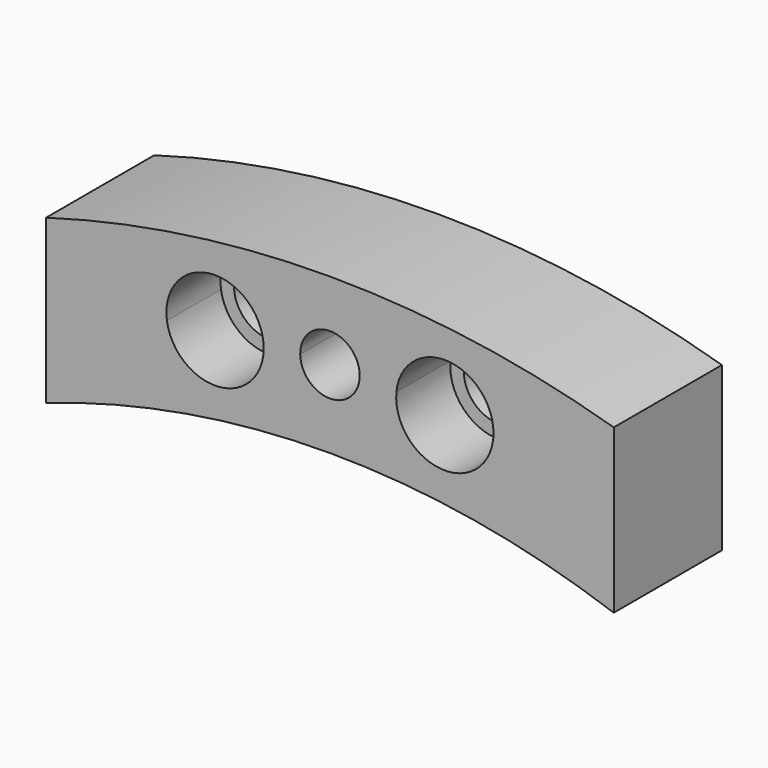
from build123d import *

# Parameters (mm, degrees)
F1_DEPTH = 50
F2_DEPTH = 25


with BuildPart() as f1:
    # F0 (on Front) → F1 (new body)
    with BuildSketch(Plane.XZ):
        with BuildLine():
            ThreePointArc((60.3004275437, 340.9588258691), (82.833452945, 336.1958976151), (105, 329.9455447494))
            Line((105, 329.9455447494), (105, 360))
            ThreePointArc((105, 360), (0, 375), (-105, 360))
            Line((-105, 360), (-105, 329.9455447494))
            ThreePointArc((-105, 329.9455447494), (-82.833452945, 336.1958976151), (-60.3004275437, 340.9588258691))
            ThreePointArc((-60.3004275437, 340.9588258691), (-44.7093862816, 361.4956891559), (-24.5847162741, 345.3761054643))
            ThreePointArc((-24.5847162741, 345.3761054643), (-17.7950983093, 345.7924189108), (-10.9986121712, 346.0752707581))
            ThreePointArc((-10.9986121712, 346.0752707581), (-0.0873673767, 357.2496530373), (11, 346.25))
            ThreePointArc((11, 346.25), (10.9996530373, 346.1626326233), (10.9986121712, 346.0752707581))
            ThreePointArc((10.9986121712, 346.0752707581), (17.7950983093, 345.7924189108), (24.5847162741, 345.3761054643))
            ThreePointArc((24.5847162741, 345.3761054643), (43.3731818064, 361.6106063163), (60.5, 343.6317978593))
            ThreePointArc((60.5, 343.6317978593), (60.4500375457, 342.2915918653), (60.3004275437, 340.9588258691))
        make_face()
        with BuildLine():
            ThreePointArc((-105, 299.635194862), (0, 317.5), (105, 299.635194862))
            Line((105, 299.635194862), (105, 329.9455447494))
            ThreePointArc((105, 329.9455447494), (82.833452945, 336.1958976151), (60.3004275437, 340.9588258691))
            ThreePointArc((60.3004275437, 340.9588258691), (40.2906137184, 325.7679065626), (24.5847162741, 345.3761054643))
            ThreePointArc((24.5847162741, 345.3761054643), (17.7950983093, 345.7924189108), (10.9986121712, 346.0752707581))
            ThreePointArc((10.9986121712, 346.0752707581), (0, 335.25), (-10.9986121712, 346.0752707581))
            ThreePointArc((-10.9986121712, 346.0752707581), (-17.7950983093, 345.7924189108), (-24.5847162741, 345.3761054643))
            ThreePointArc((-24.5847162741, 345.3761054643), (-24.521191543, 344.5049796657), (-24.5, 343.6317978593))
            ThreePointArc((-24.5, 343.6317978593), (-41.159794006, 325.6817603135), (-60.3004275437, 340.9588258691))
            ThreePointArc((-60.3004275437, 340.9588258691), (-82.833452945, 336.1958976151), (-105, 329.9455447494))
            Line((-105, 329.9455447494), (-105, 299.635194862))
        make_face()
        with BuildLine():
            ThreePointArc((-24.5847162741, 345.3761054643), (-44.7093862816, 361.4956891559), (-60.3004275437, 340.9588258691))
            ThreePointArc((-60.3004275437, 340.9588258691), (-57.8364575566, 341.3854224733), (-55.3694709553, 341.7942132133))
            ThreePointArc((-55.3694709553, 341.7942132133), (-44.09566787, 356.5334971291), (-29.5706194929, 344.9849865759))
            ThreePointArc((-29.5706194929, 344.9849865759), (-27.0783740558, 345.1895481594), (-24.5847162741, 345.3761054643))
        make_face()
        with BuildLine():
            ThreePointArc((-55.3694709553, 341.7942132133), (-57.8364575566, 341.3854224733), (-60.3004275437, 340.9588258691))
            ThreePointArc((-60.3004275437, 340.9588258691), (-41.159794006, 325.6817603135), (-24.5, 343.6317978593))
            ThreePointArc((-24.5, 343.6317978593), (-24.521191543, 344.5049796657), (-24.5847162741, 345.3761054643))
            ThreePointArc((-24.5847162741, 345.3761054643), (-27.0783740558, 345.1895481594), (-29.5706194929, 344.9849865759))
            ThreePointArc((-29.5706194929, 344.9849865759), (-29.5176668778, 344.3093129543), (-29.5, 343.6317978593))
            ThreePointArc((-29.5, 343.6317978593), (-41.5788926281, 330.6644711799), (-55.3694709553, 341.7942132133))
        make_face()
        with BuildLine():
            ThreePointArc((55.3694709553, 341.7942132133), (57.8364575566, 341.3854224733), (60.3004275437, 340.9588258691))
            ThreePointArc((60.3004275437, 340.9588258691), (60.4500375457, 342.2915918653), (60.5, 343.6317978593))
            ThreePointArc((60.5, 343.6317978593), (43.3731818064, 361.6106063163), (24.5847162741, 345.3761054643))
            ThreePointArc((24.5847162741, 345.3761054643), (27.0783740558, 345.1895481594), (29.5706194929, 344.9849865759))
            ThreePointArc((29.5706194929, 344.9849865759), (43.177515095, 356.6141309815), (55.5, 343.6317978593))
            ThreePointArc((55.5, 343.6317978593), (55.4673266794, 342.7106904874), (55.3694709553, 341.7942132133))
        make_face()
        with BuildLine():
            ThreePointArc((24.5847162741, 345.3761054643), (40.2906137184, 325.7679065626), (60.3004275437, 340.9588258691))
            ThreePointArc((60.3004275437, 340.9588258691), (57.8364575566, 341.3854224733), (55.3694709553, 341.7942132133))
            ThreePointArc((55.3694709553, 341.7942132133), (40.90433213, 330.7300985895), (29.5706194929, 344.9849865759))
            ThreePointArc((29.5706194929, 344.9849865759), (27.0783740558, 345.1895481594), (24.5847162741, 345.3761054643))
        make_face()
    extrude(amount=-F1_DEPTH)

    # F0 (on Front) → F2 (cut)
    with BuildSketch(Plane.XZ):
        with BuildLine():
            ThreePointArc((-24.5847162741, 345.3761054643), (-44.7093862816, 361.4956891559), (-60.3004275437, 340.9588258691))
            ThreePointArc((-60.3004275437, 340.9588258691), (-57.8364575566, 341.3854224733), (-55.3694709553, 341.7942132133))
            ThreePointArc((-55.3694709553, 341.7942132133), (-44.09566787, 356.5334971291), (-29.5706194929, 344.9849865759))
            ThreePointArc((-29.5706194929, 344.9849865759), (-27.0783740558, 345.1895481594), (-24.5847162741, 345.3761054643))
        make_face()
        with BuildLine():
            ThreePointArc((-55.3694709553, 341.7942132133), (-57.8364575566, 341.3854224733), (-60.3004275437, 340.9588258691))
            ThreePointArc((-60.3004275437, 340.9588258691), (-41.159794006, 325.6817603135), (-24.5, 343.6317978593))
            ThreePointArc((-24.5, 343.6317978593), (-24.521191543, 344.5049796657), (-24.5847162741, 345.3761054643))
            ThreePointArc((-24.5847162741, 345.3761054643), (-27.0783740558, 345.1895481594), (-29.5706194929, 344.9849865759))
            ThreePointArc((-29.5706194929, 344.9849865759), (-29.5176668778, 344.3093129543), (-29.5, 343.6317978593))
            ThreePointArc((-29.5, 343.6317978593), (-41.5788926281, 330.6644711799), (-55.3694709553, 341.7942132133))
        make_face()
        with BuildLine():
            ThreePointArc((55.3694709553, 341.7942132133), (57.8364575566, 341.3854224733), (60.3004275437, 340.9588258691))
            ThreePointArc((60.3004275437, 340.9588258691), (60.4500375457, 342.2915918653), (60.5, 343.6317978593))
            ThreePointArc((60.5, 343.6317978593), (43.3731818064, 361.6106063163), (24.5847162741, 345.3761054643))
            ThreePointArc((24.5847162741, 345.3761054643), (27.0783740558, 345.1895481594), (29.5706194929, 344.9849865759))
            ThreePointArc((29.5706194929, 344.9849865759), (43.177515095, 356.6141309815), (55.5, 343.6317978593))
            ThreePointArc((55.5, 343.6317978593), (55.4673266794, 342.7106904874), (55.3694709553, 341.7942132133))
        make_face()
        with BuildLine():
            ThreePointArc((24.5847162741, 345.3761054643), (40.2906137184, 325.7679065626), (60.3004275437, 340.9588258691))
            ThreePointArc((60.3004275437, 340.9588258691), (57.8364575566, 341.3854224733), (55.3694709553, 341.7942132133))
            ThreePointArc((55.3694709553, 341.7942132133), (40.90433213, 330.7300985895), (29.5706194929, 344.9849865759))
            ThreePointArc((29.5706194929, 344.9849865759), (27.0783740558, 345.1895481594), (24.5847162741, 345.3761054643))
        make_face()
    extrude(amount=-F2_DEPTH, mode=Mode.SUBTRACT)


solid = f1.part
